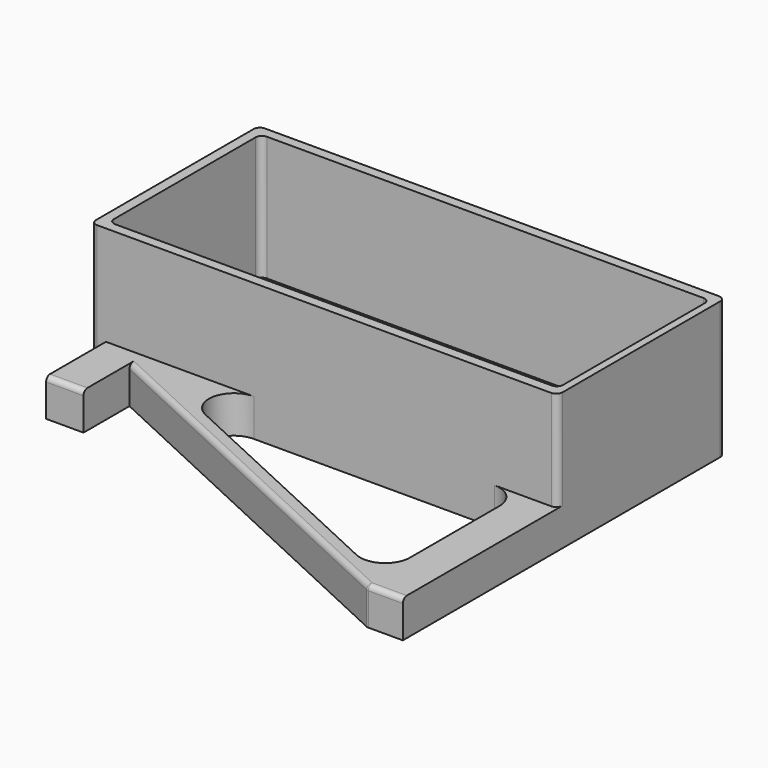
from build123d import *

# Parameters (mm, degrees)
F1_DEPTH     = 55
F2_DEPTH     = 5
F3_DEPTH     = 15
F4_DEPTH     = 15
F5_R         = 2
F6_T1_DEPTH  = 14.1054111362
F6_T6_DEPTH  = 2
F6_T12_DEPTH = 171.8572508491
F7_R         = 2


# Not quite as in the source:
# - a fillet or chamfer that OpenCascade refuses, or shapes differently, is made with other operations: its cross-section is extruded or revolved along the edge and cut away or added
# - a feature names something its author has since deleted; it is built from what else it names


with BuildPart() as f1:
    # F0 (on Top) → F1 (new body)
    with BuildSketch(Plane.XY):
        with BuildLine():
            ThreePointArc((93, 77.5), (92.267766953, 79.267766953), (90.5, 80))
            Line((90.5, 80), (36.5, 80))
            Line((36.5, 80), (24.5, 80))
            Line((24.5, 80), (19, 80))
            Line((19, 80), (-7, 80))
            Line((-7, 80), (-12.5, 80))
            Line((-12.5, 80), (-24.5, 80))
            Line((-24.5, 80), (-74, 80))
            Line((-74, 80), (-91.5, 80))
            ThreePointArc((-91.5, 80), (-93.267766953, 79.267766953), (-94, 77.5))
            Line((-94, 77.5), (-94, 76))
            Line((-94, 76), (-94, 0))
            Line((-94, 0), (-94, -1.5))
            ThreePointArc((-94, -1.5), (-93.267766953, -3.267766953), (-91.5, -4))
            Line((-91.5, -4), (-88, -4))
            Line((-88, -4), (-73, -4))
            Line((-73, -4), (-28.6959191337, -4))
            Line((-28.6959191337, -4), (67.7072161436, -4))
            Line((67.7072161436, -4), (88, -4))
            Line((88, -4), (90.5, -4))
            ThreePointArc((90.5, -4), (92.267766953, -3.267766953), (93, -1.5))
            Line((93, -1.5), (93, 0))
            Line((93, 0), (93, 76))
            Line((93, 76), (93, 77.5))
        make_face()
        with BuildLine():
            ThreePointArc((90, 2.5), (89.267766953, 0.732233047), (87.5, 0))
            Line((87.5, 0), (-87.5, 0))
            ThreePointArc((-87.5, 0), (-89.267766953, 0.732233047), (-90, 2.5))
            Line((-90, 2.5), (-90, 73.5))
            ThreePointArc((-90, 73.5), (-89.267766953, 75.267766953), (-87.5, 76))
            Line((-87.5, 76), (87.5, 76))
            ThreePointArc((87.5, 76), (89.267766953, 75.267766953), (90, 73.5))
            Line((90, 73.5), (90, 2.5))
        make_face(mode=Mode.SUBTRACT)
    extrude(amount=F1_DEPTH)

    # F0 (on Top) → F2 (join)
    with BuildSketch(Plane.XY):
        with BuildLine():
            Line((-87.5, 0), (87.5, 0))
            ThreePointArc((87.5, 0), (89.267766953, 0.732233047), (90, 2.5))
            Line((90, 2.5), (90, 73.5))
            ThreePointArc((90, 73.5), (89.267766953, 75.267766953), (87.5, 76))
            Line((87.5, 76), (-87.5, 76))
            ThreePointArc((-87.5, 76), (-89.267766953, 75.267766953), (-90, 73.5))
            Line((-90, 73.5), (-90, 2.5))
            ThreePointArc((-90, 2.5), (-89.267766953, 0.732233047), (-87.5, 0))
        make_face()
        with BuildLine():
            Line((-77.5, 66), (77.5, 66))
            ThreePointArc((77.5, 66), (79.267766953, 65.267766953), (80, 63.5))
            Line((80, 63.5), (80, 12.5))
            ThreePointArc((80, 12.5), (79.267766953, 10.732233047), (77.5, 10))
            Line((77.5, 10), (-77.5, 10))
            ThreePointArc((-77.5, 10), (-79.267766953, 10.732233047), (-80, 12.5))
            Line((-80, 12.5), (-80, 63.5))
            ThreePointArc((-80, 63.5), (-79.267766953, 65.267766953), (-77.5, 66))
        make_face(mode=Mode.SUBTRACT)
        with BuildLine():
            Line((-24.5, 80), (-12.5, 80))
            Line((-12.5, 80), (-12.5, 89.5))
            ThreePointArc((-12.5, 89.5), (-13.232233047, 91.267766953), (-15, 92))
            Line((-15, 92), (-22, 92))
            ThreePointArc((-22, 92), (-23.767766953, 91.267766953), (-24.5, 89.5))
            Line((-24.5, 89.5), (-24.5, 80))
        make_face()
        with BuildLine():
            Line((-7, 80), (19, 80))
            Line((19, 80), (19, 89.5))
            ThreePointArc((19, 89.5), (18.267766953, 91.267766953), (16.5, 92))
            Line((16.5, 92), (-4.5, 92))
            ThreePointArc((-4.5, 92), (-6.267766953, 91.267766953), (-7, 89.5))
            Line((-7, 89.5), (-7, 80))
        make_face()
        with BuildLine():
            Line((24.5, 80), (36.5, 80))
            Line((36.5, 80), (36.5, 89.5))
            ThreePointArc((36.5, 89.5), (35.767766953, 91.267766953), (34, 92))
            Line((34, 92), (27, 92))
            ThreePointArc((27, 92), (25.232233047, 91.267766953), (24.5, 89.5))
            Line((24.5, 89.5), (24.5, 80))
        make_face()
    extrude(amount=F2_DEPTH)

    # F0 (on Top) → F3 (join)
    with BuildSketch(Plane.XY):
        with BuildLine():
            Line((93, -81.5), (93, -1.5))
            ThreePointArc((93, -1.5), (92.267766953, -3.267766953), (90.5, -4))
            Line((90.5, -4), (88, -4))
            Line((88, -4), (67.7072161436, -4))
            ThreePointArc((67.7072161436, -4), (74.7782839555, -6.9289321881), (77.7072161436, -14))
            Line((77.7072161436, -14), (77.7072161436, -58.7379819401))
            ThreePointArc((77.7072161436, -58.7379819401), (73.0879609173, -67.1669549309), (63.4976990076, -67.8088124137))
            Line((63.4976990076, -67.8088124137), (-32.9054362697, -23.0708304737))
            ThreePointArc((-32.9054362697, -23.0708304737), (-38.4608642113, -11.8445771571), (-28.6959191337, -4))
            Line((-28.6959191337, -4), (-73, -4))
            Line((-73, -4), (-73, -10.9733034172))
            Line((-73, -10.9733034172), (78.7072161436, -81.5))
            Line((78.7072161436, -81.5), (93, -81.5))
        make_face()
    extrude(amount=F3_DEPTH)

    # F0 (on Top) → F4 (join)
    with BuildSketch(Plane.XY):
        Polygon((-88, -4), (-73, -10.9733034172), (-73, -4), align=None)
        Polygon((-73, -34), (-73, -10.9733034172), (-88, -4), (-88, -34), align=None)
    extrude(amount=F4_DEPTH)

    # F5
    f5_edges = [f1.edges().sort_by_distance(p)[0] for p in [
        (85.853608, -81.5, 15),
    ]]
    fillet(f5_edges, radius=F5_R)

    # F6: fillet of radius 2 on 1 edges, made by hand

    # F6_s2 → F6_t1 (cut)
    with BuildSketch(Plane.XY.offset(-1.1054111362)):
        with BuildLine():
            ThreePointArc((78.3062611352, -81.3136012713), (78.7176414075, -81.4528444053), (79.1493805981, -81.5))
            Line((79.1493805981, -81.5), (78.7072161436, -81.5))
            Line((78.7072161436, -81.5), (78.3062611352, -81.3136012713))
        make_face()
    extrude(amount=F6_T1_DEPTH, mode=Mode.SUBTRACT)


with BuildPart() as f6_tool4:
    # F6_s5 → F6_t6 (new body)
    with BuildSketch(Plane.XY.offset(13)):
        Polygon((79.1493805981, -79.5), (78.3062611352, -81.3136012713), (78.7072161436, -81.5), (79.1493805981, -81.5), align=None)
    extrude(amount=F6_T6_DEPTH)

    # F6_s7 → F6_t8 (revolve, cut)
    with BuildSketch(Plane(origin=(79.1493805981, -79.5, 13), x_dir=(0.2158695953, 0.9764222027, 0), z_dir=(0.9764222027, -0.2158695953, 0))):
        with BuildLine():
            ThreePointArc((0, -2), (2, 0), (0, 2))
            Line((0, 2), (0, -2))
        make_face()
    revolve(axis=Axis((79.1493805981, -79.5, 13), (0, 0, 1)), mode=Mode.SUBTRACT)


with BuildPart() as f1_1:
    add(f1.part)

    # F6_t3: cut F6_tool4
    add(f6_tool4.part, mode=Mode.SUBTRACT)


with BuildPart() as f6_tool10:
    # F6_s11 → F6_t12 (new body)
    with BuildSketch(Plane(origin=(-60.3662112187, 28.0634604648, 0), x_dir=(0, 0, 1), z_dir=(0.9068006357, -0.4215597314, 0))):
        with BuildLine():
            ThreePointArc((15, 38.724458908), (14.4142135624, 40.1386724704), (13, 40.724458908))
            Line((13, 40.724458908), (15, 40.724458908))
            Line((15, 40.724458908), (15, 38.724458908))
        make_face()
    extrude(amount=F6_T12_DEPTH)

    split(bisect_by=Plane.YZ.offset(-73), keep=Keep.TOP)


with BuildPart() as f1_2:
    add(f1_1.part)

    # F6_t9: cut F6_tool10
    add(f6_tool10.part, mode=Mode.SUBTRACT)

    # F7
    f7_edges = [f1_2.edges().sort_by_distance(p)[0] for p in [
        (-80.5, -34, 15),
    ]]
    fillet(f7_edges, radius=F7_R)


solid = f1_2.part
